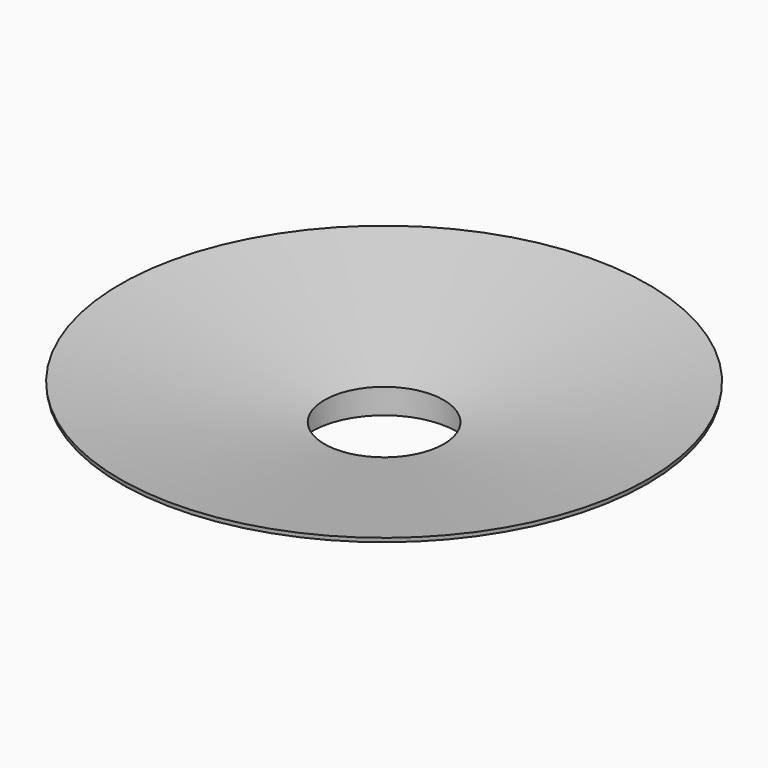
from build123d import *

# Parameters (mm, degrees)
F0_W = 1.1887382716
F0_H = 8.2106888294


# Not quite as in the source:
# - the program builds the solid bodies; features that only make, move or delete a surface that nothing else refers to are left out


with BuildPart() as f2:
    # F0 (on Front) → F2 (revolve)
    with BuildSketch(Plane.XZ):
        with Locations((20.5420861021, 4.1053444147)):
            Rectangle(F0_W, F0_H)
    revolve(axis=Axis((0, 0, 14.6341603249), (0, 0, 1)))


with BuildPart() as f4:
    # F3 (on Front) → F4 (revolve)
    with BuildSketch(Plane.XZ):
        with BuildLine():
            add(Edge.make_bspline(
                [(20.3322526067, 8.2946820185), (19.2627200389, 8.4468284836), (18.1931874711, 8.5989749487), (16.4470637122, 8.7455055095)],
                knots=[0, 0, 0, 0, 0.3276532475, 0.3276532475, 0.3276532475, 0.3276532475], degree=3))
            Line((20.3322526067, 8.2946820185), (72.5994333625, 17.368843779))
            Line((72.5994333625, 17.368843779), (72.7768065665, 18.5249730683))
            Line((72.7768065665, 18.5249730683), (16.4470637122, 8.7455055095))
        make_face()
    revolve(axis=Axis((0, 0, 14.6341603249), (0, 0, 1)))


solid = Compound([f2.part, f4.part])
